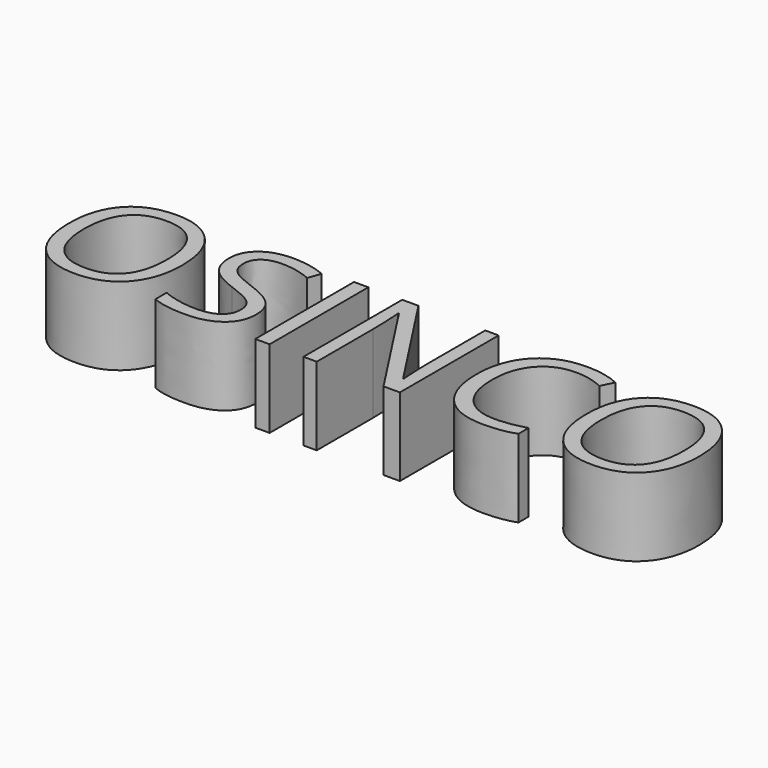
from build123d import *

# Parameters (mm, degrees)
F1_TEXT_SIZE = 22.1407351394
F2_DEPTH     = 10


# Not quite as in the source:
# - Text() gives the source's letters only with a copy of the font that has no kerning and outlines rounded to 1/6400 em; it was checked with that copy


with BuildPart() as f2:
    # F1 (on face) → F2 (new body)
    with BuildSketch(Plane.XY):
        with Locations((11.497721076, -17.9084669799)):
            Text('OSINCO', F1_TEXT_SIZE, font='Open Sans', text_align=(TextAlign.LEFT, TextAlign.BOTTOM))
    extrude(amount=F2_DEPTH)


solid = f2.part
